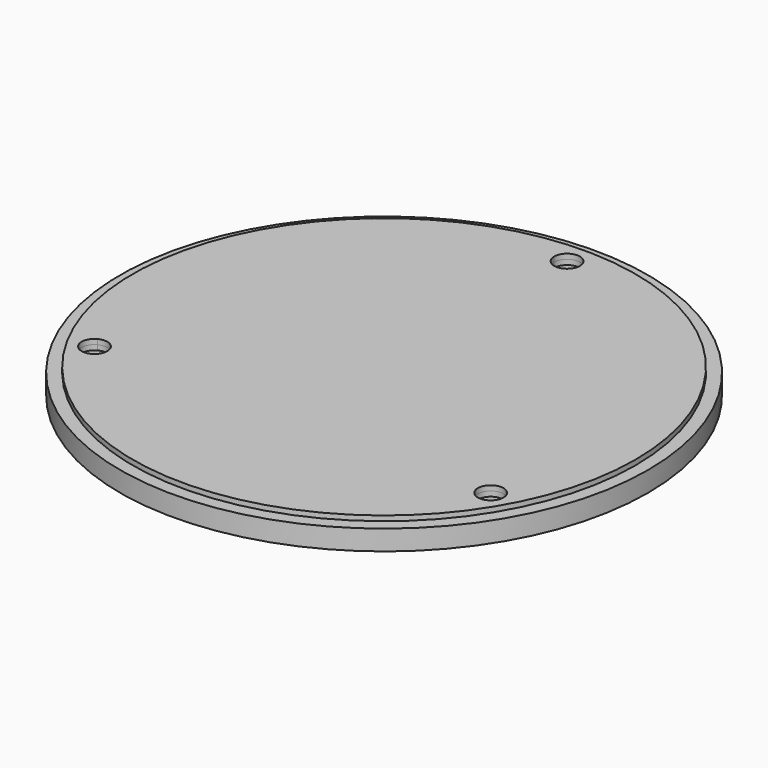
from build123d import *
from build123d import SkipClean  # not in build123d's __all__

# Parameters (mm, degrees)
F0_R     = 25
F1_DEPTH = 0.5
F0_R_2   = 26.25
F2_DEPTH = 2
F3_DEPTH = 0.5


with BuildPart() as f1:
    # F0 (on Top) → F1 (new body)
    with BuildSketch(Plane.XY):
        Circle(F0_R)
        with BuildLine():
            ThreePointArc((1.998066932, 22.6620879121), (16.7782377308, 15.3640241684), (22.75, 0))
            ThreePointArc((22.75, 0), (22.2123921898, -4.9165163688), (20.6249773007, -9.6006672345))
            ThreePointArc((20.6249773007, -9.6006672345), (21.4117268371, -10.3371654104), (21.7020779361, -11.375))
            ThreePointArc((21.7020779361, -11.375), (20.6637600211, -13.12861557), (18.6269103687, -13.0614206776))
            ThreePointArc((18.6269103687, -13.0614206776), (0, -22.75), (-18.6269103687, -13.0614206776))
            ThreePointArc((-18.6269103687, -13.0614206776), (-21.4341287437, -12.375), (-20.6249773007, -9.6006672345))
            ThreePointArc((-20.6249773007, -9.6006672345), (-19.7020779361, 11.375), (-1.998066932, 22.6620879121))
            ThreePointArc((-1.998066932, 22.6620879121), (-0.0439666691, 24.7495166746), (2, 22.75))
            ThreePointArc((2, 22.75), (1.9995166746, 22.7060333309), (1.998066932, 22.6620879121))
        make_face(mode=Mode.SUBTRACT)
        with BuildLine():
            ThreePointArc((20.6249773007, -9.6006672345), (22.2123921898, -4.9165163688), (22.75, 0))
            ThreePointArc((22.75, 0), (16.7782377308, 15.3640241684), (1.998066932, 22.6620879121))
            ThreePointArc((1.998066932, 22.6620879121), (0, 20.75), (-1.998066932, 22.6620879121))
            ThreePointArc((-1.998066932, 22.6620879121), (-19.7020779361, 11.375), (-20.6249773007, -9.6006672345))
            ThreePointArc((-20.6249773007, -9.6006672345), (-18.6642433465, -9.665351099), (-17.7020779361, -11.375))
            ThreePointArc((-17.7020779361, -11.375), (-17.9484623661, -12.336682085), (-18.6269103687, -13.0614206776))
            ThreePointArc((-18.6269103687, -13.0614206776), (0, -22.75), (18.6269103687, -13.0614206776))
            ThreePointArc((18.6269103687, -13.0614206776), (17.9700271285, -10.375), (20.6249773007, -9.6006672345))
        make_face()
        with BuildLine():
            ThreePointArc((-20.3083862198, -10.2533872036), (-20.4692836493, -9.9282892225), (-20.6249773007, -9.6006672345))
            ThreePointArc((-20.6249773007, -9.6006672345), (-21.4341287437, -12.375), (-18.6269103687, -13.0614206776))
            ThreePointArc((-18.6269103687, -13.0614206776), (-18.8327925074, -12.7627750263), (-19.0338869031, -12.4608847744))
            ThreePointArc((-19.0338869031, -12.4608847744), (-20.8062603259, -12.0125), (-20.3083862198, -10.2533872036))
        make_face()
        with BuildLine():
            ThreePointArc((21.7020779361, -11.375), (21.4117268371, -10.3371654104), (20.6249773007, -9.6006672345))
            ThreePointArc((20.6249773007, -9.6006672345), (20.4692836493, -9.9282892225), (20.3083862198, -10.2533872036))
            ThreePointArc((20.3083862198, -10.2533872036), (20.797219037, -10.7220903821), (20.9770779361, -11.375))
            ThreePointArc((20.9770779361, -11.375), (20.3240431413, -12.4880068659), (19.0338869031, -12.4608847744))
            ThreePointArc((19.0338869031, -12.4608847744), (18.8327925074, -12.7627750263), (18.6269103687, -13.0614206776))
            ThreePointArc((18.6269103687, -13.0614206776), (20.6637600211, -13.12861557), (21.7020779361, -11.375))
        make_face()
        with BuildLine():
            ThreePointArc((1.2744993168, 22.714271978), (1.6364911418, 22.6910642488), (1.998066932, 22.6620879121))
            ThreePointArc((1.998066932, 22.6620879121), (1.9995166746, 22.7060333309), (2, 22.75))
            ThreePointArc((2, 22.75), (-0.0439666691, 24.7495166746), (-1.998066932, 22.6620879121))
            ThreePointArc((-1.998066932, 22.6620879121), (-1.6364911418, 22.6910642488), (-1.2744993168, 22.714271978))
            ThreePointArc((-1.2744993168, 22.714271978), (-0.017865765, 24.024874823), (1.275, 22.75))
            ThreePointArc((1.275, 22.75), (1.274874823, 22.732134235), (1.2744993168, 22.714271978))
        make_face()
        with BuildLine():
            ThreePointArc((-17.7020779361, -11.375), (-18.6642433465, -9.665351099), (-20.6249773007, -9.6006672345))
            ThreePointArc((-20.6249773007, -9.6006672345), (-20.4692836493, -9.9282892225), (-20.3083862198, -10.2533872036))
            ThreePointArc((-20.3083862198, -10.2533872036), (-19.0491683182, -10.2798588991), (-18.4270779361, -11.375))
            ThreePointArc((-18.4270779361, -11.375), (-18.5890710702, -11.9969652052), (-19.0338869031, -12.4608847744))
            ThreePointArc((-19.0338869031, -12.4608847744), (-18.8327925074, -12.7627750263), (-18.6269103687, -13.0614206776))
            ThreePointArc((-18.6269103687, -13.0614206776), (-17.9484623661, -12.336682085), (-17.7020779361, -11.375))
        make_face()
        with BuildLine():
            ThreePointArc((20.3083862198, -10.2533872036), (20.4692836493, -9.9282892225), (20.6249773007, -9.6006672345))
            ThreePointArc((20.6249773007, -9.6006672345), (17.9700271285, -10.375), (18.6269103687, -13.0614206776))
            ThreePointArc((18.6269103687, -13.0614206776), (18.8327925074, -12.7627750263), (19.0338869031, -12.4608847744))
            ThreePointArc((19.0338869031, -12.4608847744), (18.5978955463, -10.7375), (20.3083862198, -10.2533872036))
        make_face()
        with BuildLine():
            ThreePointArc((-1.998066932, 22.6620879121), (0, 20.75), (1.998066932, 22.6620879121))
            ThreePointArc((1.998066932, 22.6620879121), (1.6364911418, 22.6910642488), (1.2744993168, 22.714271978))
            ThreePointArc((1.2744993168, 22.714271978), (0, 21.475), (-1.2744993168, 22.714271978))
            ThreePointArc((-1.2744993168, 22.714271978), (-1.6364911418, 22.6910642488), (-1.998066932, 22.6620879121))
        make_face()
    extrude(amount=F1_DEPTH)

    # F0 (on Top) → F2 (join)
    with BuildSketch(Plane.XY):
        Circle(F0_R_2)
        Circle(F0_R, mode=Mode.SUBTRACT)
        Circle(F0_R)
        with BuildLine():
            ThreePointArc((1.998066932, 22.6620879121), (16.7782377308, 15.3640241684), (22.75, 0))
            ThreePointArc((22.75, 0), (22.2123921898, -4.9165163688), (20.6249773007, -9.6006672345))
            ThreePointArc((20.6249773007, -9.6006672345), (21.4117268371, -10.3371654104), (21.7020779361, -11.375))
            ThreePointArc((21.7020779361, -11.375), (20.6637600211, -13.12861557), (18.6269103687, -13.0614206776))
            ThreePointArc((18.6269103687, -13.0614206776), (0, -22.75), (-18.6269103687, -13.0614206776))
            ThreePointArc((-18.6269103687, -13.0614206776), (-21.4341287437, -12.375), (-20.6249773007, -9.6006672345))
            ThreePointArc((-20.6249773007, -9.6006672345), (-19.7020779361, 11.375), (-1.998066932, 22.6620879121))
            ThreePointArc((-1.998066932, 22.6620879121), (-0.0439666691, 24.7495166746), (2, 22.75))
            ThreePointArc((2, 22.75), (1.9995166746, 22.7060333309), (1.998066932, 22.6620879121))
        make_face(mode=Mode.SUBTRACT)
        with BuildLine():
            ThreePointArc((20.6249773007, -9.6006672345), (22.2123921898, -4.9165163688), (22.75, 0))
            ThreePointArc((22.75, 0), (16.7782377308, 15.3640241684), (1.998066932, 22.6620879121))
            ThreePointArc((1.998066932, 22.6620879121), (0, 20.75), (-1.998066932, 22.6620879121))
            ThreePointArc((-1.998066932, 22.6620879121), (-19.7020779361, 11.375), (-20.6249773007, -9.6006672345))
            ThreePointArc((-20.6249773007, -9.6006672345), (-18.6642433465, -9.665351099), (-17.7020779361, -11.375))
            ThreePointArc((-17.7020779361, -11.375), (-17.9484623661, -12.336682085), (-18.6269103687, -13.0614206776))
            ThreePointArc((-18.6269103687, -13.0614206776), (0, -22.75), (18.6269103687, -13.0614206776))
            ThreePointArc((18.6269103687, -13.0614206776), (17.9700271285, -10.375), (20.6249773007, -9.6006672345))
        make_face()
    extrude(amount=-F2_DEPTH)

    # F0 (on Top) → F3 (join)
    with BuildSketch(Plane.XY):
        with BuildLine():
            ThreePointArc((1.2744993168, 22.714271978), (1.6364911418, 22.6910642488), (1.998066932, 22.6620879121))
            ThreePointArc((1.998066932, 22.6620879121), (1.9995166746, 22.7060333309), (2, 22.75))
            ThreePointArc((2, 22.75), (-0.0439666691, 24.7495166746), (-1.998066932, 22.6620879121))
            ThreePointArc((-1.998066932, 22.6620879121), (-1.6364911418, 22.6910642488), (-1.2744993168, 22.714271978))
            ThreePointArc((-1.2744993168, 22.714271978), (-0.017865765, 24.024874823), (1.275, 22.75))
            ThreePointArc((1.275, 22.75), (1.274874823, 22.732134235), (1.2744993168, 22.714271978))
        make_face()
        with BuildLine():
            ThreePointArc((-1.998066932, 22.6620879121), (0, 20.75), (1.998066932, 22.6620879121))
            ThreePointArc((1.998066932, 22.6620879121), (1.6364911418, 22.6910642488), (1.2744993168, 22.714271978))
            ThreePointArc((1.2744993168, 22.714271978), (0, 21.475), (-1.2744993168, 22.714271978))
            ThreePointArc((-1.2744993168, 22.714271978), (-1.6364911418, 22.6910642488), (-1.998066932, 22.6620879121))
        make_face()
        with BuildLine():
            ThreePointArc((-20.3083862198, -10.2533872036), (-20.4692836493, -9.9282892225), (-20.6249773007, -9.6006672345))
            ThreePointArc((-20.6249773007, -9.6006672345), (-21.4341287437, -12.375), (-18.6269103687, -13.0614206776))
            ThreePointArc((-18.6269103687, -13.0614206776), (-18.8327925074, -12.7627750263), (-19.0338869031, -12.4608847744))
            ThreePointArc((-19.0338869031, -12.4608847744), (-20.8062603259, -12.0125), (-20.3083862198, -10.2533872036))
        make_face()
        with BuildLine():
            ThreePointArc((-17.7020779361, -11.375), (-18.6642433465, -9.665351099), (-20.6249773007, -9.6006672345))
            ThreePointArc((-20.6249773007, -9.6006672345), (-20.4692836493, -9.9282892225), (-20.3083862198, -10.2533872036))
            ThreePointArc((-20.3083862198, -10.2533872036), (-19.0491683182, -10.2798588991), (-18.4270779361, -11.375))
            ThreePointArc((-18.4270779361, -11.375), (-18.5890710702, -11.9969652052), (-19.0338869031, -12.4608847744))
            ThreePointArc((-19.0338869031, -12.4608847744), (-18.8327925074, -12.7627750263), (-18.6269103687, -13.0614206776))
            ThreePointArc((-18.6269103687, -13.0614206776), (-17.9484623661, -12.336682085), (-17.7020779361, -11.375))
        make_face()
        with BuildLine():
            ThreePointArc((20.3083862198, -10.2533872036), (20.4692836493, -9.9282892225), (20.6249773007, -9.6006672345))
            ThreePointArc((20.6249773007, -9.6006672345), (17.9700271285, -10.375), (18.6269103687, -13.0614206776))
            ThreePointArc((18.6269103687, -13.0614206776), (18.8327925074, -12.7627750263), (19.0338869031, -12.4608847744))
            ThreePointArc((19.0338869031, -12.4608847744), (18.5978955463, -10.7375), (20.3083862198, -10.2533872036))
        make_face()
        with BuildLine():
            ThreePointArc((21.7020779361, -11.375), (21.4117268371, -10.3371654104), (20.6249773007, -9.6006672345))
            ThreePointArc((20.6249773007, -9.6006672345), (20.4692836493, -9.9282892225), (20.3083862198, -10.2533872036))
            ThreePointArc((20.3083862198, -10.2533872036), (20.797219037, -10.7220903821), (20.9770779361, -11.375))
            ThreePointArc((20.9770779361, -11.375), (20.3240431413, -12.4880068659), (19.0338869031, -12.4608847744))
            ThreePointArc((19.0338869031, -12.4608847744), (18.8327925074, -12.7627750263), (18.6269103687, -13.0614206776))
            ThreePointArc((18.6269103687, -13.0614206776), (20.6637600211, -13.12861557), (21.7020779361, -11.375))
        make_face()
    with SkipClean():  # cleaning this boolean's faces spoils the solid; the shape is the same uncleaned
        extrude(amount=-F3_DEPTH)


solid = f1.part
